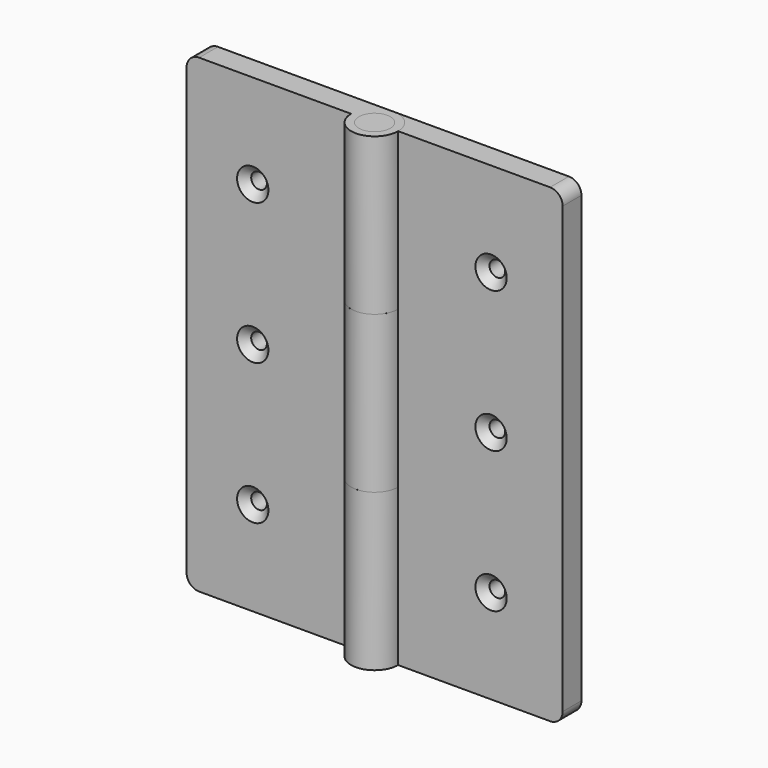
from build123d import *

# Parameters (mm, degrees)
F0_R             = 6.35
F1_DEPTH         = 95.25
F2_DEPTH         = 31.75
F3_DEPTH         = 31.75
F4_DEPTH         = 95.25
F6_D             = 6.35
F6_CSINK_D       = 12.7
F6_CSINK_ANGLE   = 90
F6_2_D           = 6.35
F6_2_CSINK_D     = 12.7
F6_2_CSINK_ANGLE = 90
F7_DEPTH         = 95.25
F8_R             = 5.08
F8_2_R           = 5.08


with BuildPart() as f1:
    # F0 (on Top) → F1 (new body, symmetric)
    with BuildSketch(Plane.XY):
        with BuildLine():
            ThreePointArc((-9.525, 0), (-6.7351920908, 6.7351920908), (0, 9.525))
            Line((0, 9.525), (-76.2, 9.525))
            Line((-76.2, 9.525), (-76.2, 0))
            Line((-76.2, 0), (-9.525, 0))
        make_face()
        with BuildLine():
            ThreePointArc((-9.525, 0), (0, -9.525), (9.525, 0))
            ThreePointArc((9.525, 0), (6.7351920908, 6.7351920908), (0, 9.525))
            ThreePointArc((0, 9.525), (-6.7351920908, 6.7351920908), (-9.525, 0))
        make_face()
        Circle(F0_R, mode=Mode.SUBTRACT)
    extrude(amount=F1_DEPTH, both=True)

    # F0 (on Top) → F2 (cut, symmetric)
    with BuildSketch(Plane.XY):
        with BuildLine():
            ThreePointArc((-9.525, 0), (0, -9.525), (9.525, 0))
            ThreePointArc((9.525, 0), (6.7351920908, 6.7351920908), (0, 9.525))
            ThreePointArc((0, 9.525), (-6.7351920908, 6.7351920908), (-9.525, 0))
        make_face()
        Circle(F0_R, mode=Mode.SUBTRACT)
    extrude(amount=F2_DEPTH, both=True, mode=Mode.SUBTRACT)

    # F6 (through all)
    with Locations(Plane.XZ):
        with Locations((-49.3769919423, 57.15), (47.2024205584, 57.15), (47.2024205584, 0), (-49.3769919423, 0), (-49.3769919423, -57.15), (47.2024205584, -57.15)):
            CounterSinkHole(F6_D / 2, F6_CSINK_D / 2, counter_sink_angle=F6_CSINK_ANGLE)

    # F8
    f8_edges = [f1.edges().sort_by_distance(p)[0] for p in [
        (-76.2, 4.7625, -95.25),
        (-76.2, 4.7625, 95.25),
    ]]
    fillet(f8_edges, radius=F8_R)


with BuildPart() as f3:
    # F0 (on Top) → F3 (new body, symmetric)
    with BuildSketch(Plane.XY):
        with BuildLine():
            ThreePointArc((-9.525, 0), (0, -9.525), (9.525, 0))
            ThreePointArc((9.525, 0), (6.7351920908, 6.7351920908), (0, 9.525))
            ThreePointArc((0, 9.525), (-6.7351920908, 6.7351920908), (-9.525, 0))
        make_face()
        Circle(F0_R, mode=Mode.SUBTRACT)
    extrude(amount=F3_DEPTH, both=True)

    # F0 (on Top) → F4 (join, symmetric)
    with BuildSketch(Plane.XY):
        with BuildLine():
            ThreePointArc((0, 9.525), (6.7351920908, 6.7351920908), (9.525, 0))
            Line((9.525, 0), (76.2, 0))
            Line((76.2, 0), (76.2, 9.525))
            Line((76.2, 9.525), (0, 9.525))
        make_face()
    extrude(amount=F4_DEPTH, both=True)

    # F6#2 (through all)
    with Locations(Plane.XZ):
        with Locations((-49.3769919423, 57.15), (47.2024205584, 57.15), (47.2024205584, 0), (-49.3769919423, 0), (-49.3769919423, -57.15), (47.2024205584, -57.15)):
            CounterSinkHole(F6_2_D / 2, F6_2_CSINK_D / 2, counter_sink_angle=F6_2_CSINK_ANGLE)

    # F8#2
    f8_2_edges = [f3.edges().sort_by_distance(p)[0] for p in [
        (76.2, 4.7625, 95.25),
        (76.2, 4.7625, -95.25),
    ]]
    fillet(f8_2_edges, radius=F8_2_R)


with BuildPart() as f7:
    # F0 (on Top) → F7 (new body, symmetric)
    with BuildSketch(Plane.XY):
        Circle(F0_R)
    extrude(amount=F7_DEPTH, both=True)


solid = Compound([f1.part, f3.part, f7.part])
